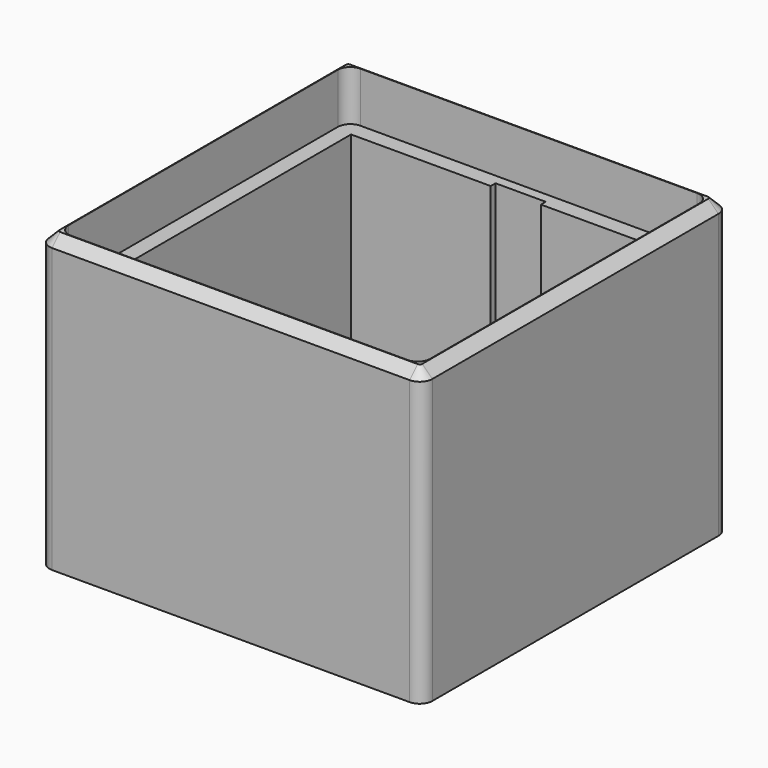
from build123d import *

# Parameters (mm, degrees)
F1_DEPTH  = 18.5547
F3_DEPTH  = 33.9344
F4_W      = 45.72
F4_H      = 45.72
F5_DEPTH  = 6.35
F6_R      = 1.5875
F7_DEPTH  = 4.7752
F8_R      = 1.5875
F9_W      = 6.35
F9_H      = 0.762
F10_DEPTH = 27.5844
F11_SIZE  = 1.27


with BuildPart() as f1:
    # F0 (on Top) → F1 (new body, symmetric)
    with BuildSketch(Plane.XY):
        with BuildLine():
            ThreePointArc((24.1935, 22.606), (23.7285320151, 23.7285320151), (22.606, 24.1935))
            Line((22.606, 24.1935), (-22.606, 24.1935))
            ThreePointArc((-22.606, 24.1935), (-23.7285320151, 23.7285320151), (-24.1935, 22.606))
            Line((-24.1935, 22.606), (-24.1935, -22.606))
            ThreePointArc((-24.1935, -22.606), (-23.7285320151, -23.7285320151), (-22.606, -24.1935))
            Line((-22.606, -24.1935), (22.606, -24.1935))
            ThreePointArc((22.606, -24.1935), (23.7285320151, -23.7285320151), (24.1935, -22.606))
            Line((24.1935, -22.606), (24.1935, 22.606))
        make_face()
    extrude(amount=F1_DEPTH, both=True)

    # F2 (on face) → F3 (cut)
    with BuildSketch(Plane.XY.offset(18.5547)):
        Polygon((20.828, -20.3835), (20.828, 20.3835), (20.828, 20.828), (20.3835, 20.828), (-20.3835, 20.828), (-20.828, 20.828), (-20.828, 20.3835), (-20.828, -20.3835), (-20.828, -20.828), (-20.3835, -20.828), (20.3835, -20.828), (20.828, -20.828), align=None)
    extrude(amount=-F3_DEPTH, mode=Mode.SUBTRACT)

    # F4 (on face) → F5 (cut)
    with BuildSketch(Plane.XY.offset(18.5547)):
        Rectangle(F4_W, F4_H)
    extrude(amount=-F5_DEPTH, mode=Mode.SUBTRACT)

    # F6 (on face) → F7 (join)
    with BuildSketch(Plane.XY.offset(-15.3797)):
        with Locations((17.4514236985, -17.4514236985)):
            Circle(F6_R)
        with Locations((-17.4514236985, -17.4514236985)):
            Circle(F6_R)
        with Locations((-17.4514236985, 17.4514236985)):
            Circle(F6_R)
        with Locations((17.4514236985, 17.4514236985)):
            Circle(F6_R)
    extrude(amount=F7_DEPTH)

    # F8
    f8_edges = [f1.edges().sort_by_distance(p)[0] for p in [
        (22.86, 22.86, 15.3797),
        (-22.86, 22.86, 15.3797),
        (-22.86, -22.86, 15.3797),
        (22.86, -22.86, 15.3797),
    ]]
    fillet(f8_edges, radius=F8_R)

    # F9 (on face) → F10 (cut, through all)
    with BuildSketch(Plane.XY.offset(12.2047)):
        with Locations((0, 21.209)):
            Rectangle(F9_W, F9_H)
        with Locations((0, -21.209)):
            Rectangle(F9_W, F9_H)
    extrude(amount=-F10_DEPTH, mode=Mode.SUBTRACT)

    # F11
    f11_edges = [f1.edges().sort_by_distance(p)[0] for p in [
        (-23.728532, 23.728532, 18.5547),
        (-24.1935, 0, 18.5547),
        (-23.728532, -23.728532, 18.5547),
        (0, -24.1935, 18.5547),
        (23.728532, -23.728532, 18.5547),
        (24.1935, 0, 18.5547),
        (0, 24.1935, 18.5547),
    ]]
    chamfer(f11_edges, length=F11_SIZE)


solid = f1.part
